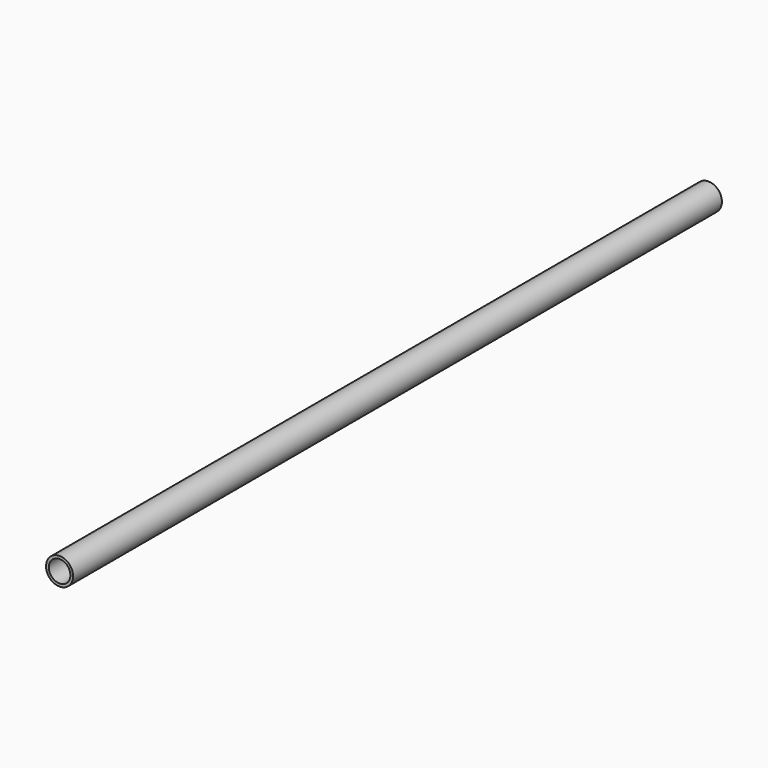
from build123d import *

# Parameters (mm, degrees)
F0_R     = 7.9375
F0_R_2   = 6.35
F2_DEPTH = 476.25


# Not quite as in the source:
# - a variable given as a bare number and used for a length is read in inches; the dataset says mm whatever the document's units were


with BuildPart() as f2:
    # F0 (on Front) → F2 (new body)
    with BuildSketch(Plane.XZ):
        Circle(F0_R)
        Circle(F0_R_2, mode=Mode.SUBTRACT)
    extrude(amount=F2_DEPTH)


solid = f2.part
